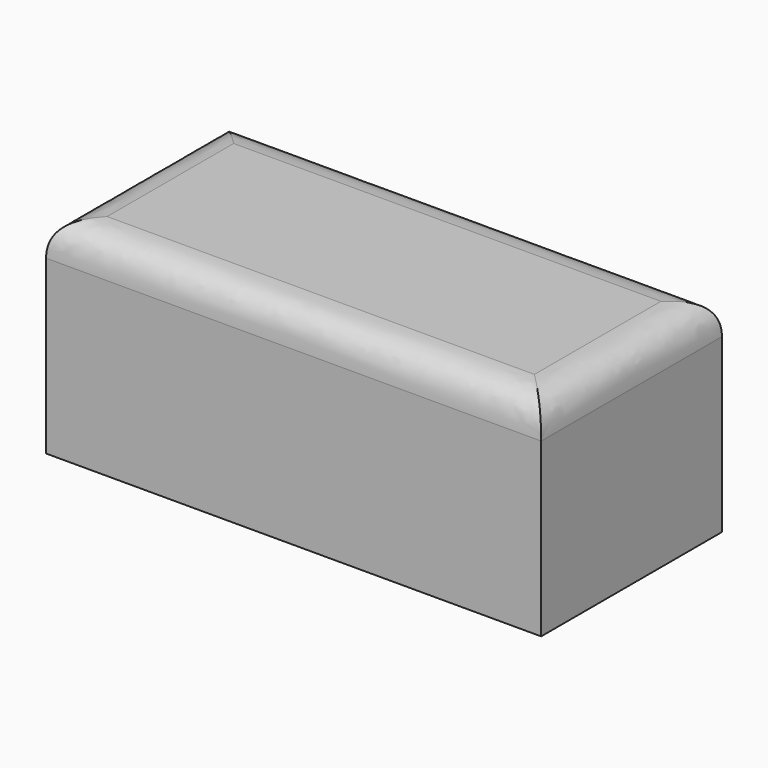
from build123d import *

# Parameters (mm, degrees)
F0_W        = 26.8767457455
F0_H        = 12.2668221593
F1_DEPTH    = 11.176
F2_T1_DEPTH = 21.4649758319
F2_T3_DEPTH = 36.0748994182


# Not quite as in the source:
# - a fillet or chamfer that OpenCascade refuses, or shapes differently, is made with other operations: its cross-section is extruded or revolved along the edge and cut away or added


with BuildPart() as f1:
    # F0 (on Top) → F1 (new body)
    with BuildSketch(Plane.XY):
        Rectangle(F0_W, F0_H)
    extrude(amount=F1_DEPTH)

    # F2: fillet of radius 1.8396307345 on 4 edges, made by hand

    # F2_s2 → F2_t1 (cut)
    with BuildSketch(Plane.XZ.offset(-10.732487916)):
        with BuildLine():
            add(Edge.make_bspline(
                [(13.4383728728, 9.3363692655), (13.4383728728, 11.176), (11.5987421382, 11.176)],
                knots=[0, 0, 0, 1, 1, 1], degree=2, weights=[1, 1, 1]))
            Line((11.5987421382, 11.176), (13.4383728728, 11.176))
            Line((13.4383728728, 11.176), (13.4383728728, 9.3363692655))
        make_face()
        with BuildLine():
            add(Edge.make_bspline(
                [(-13.4383728728, 9.3363692655), (-13.4383728728, 11.176), (-11.5987421382, 11.176)],
                knots=[0, 0, 0, 1, 1, 1], degree=2, weights=[1, 1, 1]))
            Line((-11.5987421382, 11.176), (-13.4383728728, 11.176))
            Line((-13.4383728728, 11.176), (-13.4383728728, 9.3363692655))
        make_face()
    extrude(amount=F2_T1_DEPTH, mode=Mode.SUBTRACT)

    # F2_s4 → F2_t3 (cut)
    with BuildSketch(Plane.YZ.offset(-18.0374497091)):
        with BuildLine():
            add(Edge.make_bspline(
                [(6.1334110796, 9.3363692655), (6.1334110796, 11.176), (4.2937803451, 11.176)],
                knots=[0, 0, 0, 1, 1, 1], degree=2, weights=[1, 1, 1]))
            Line((4.2937803451, 11.176), (6.1334110796, 11.176))
            Line((6.1334110796, 11.176), (6.1334110796, 9.3363692655))
        make_face()
        with BuildLine():
            add(Edge.make_bspline(
                [(-6.1334110796, 9.3363692655), (-6.1334110796, 11.176), (-4.2937803451, 11.176)],
                knots=[0, 0, 0, 1, 1, 1], degree=2, weights=[1, 1, 1]))
            Line((-4.2937803451, 11.176), (-6.1334110796, 11.176))
            Line((-6.1334110796, 11.176), (-6.1334110796, 9.3363692655))
        make_face()
    extrude(amount=F2_T3_DEPTH, mode=Mode.SUBTRACT)


solid = f1.part
